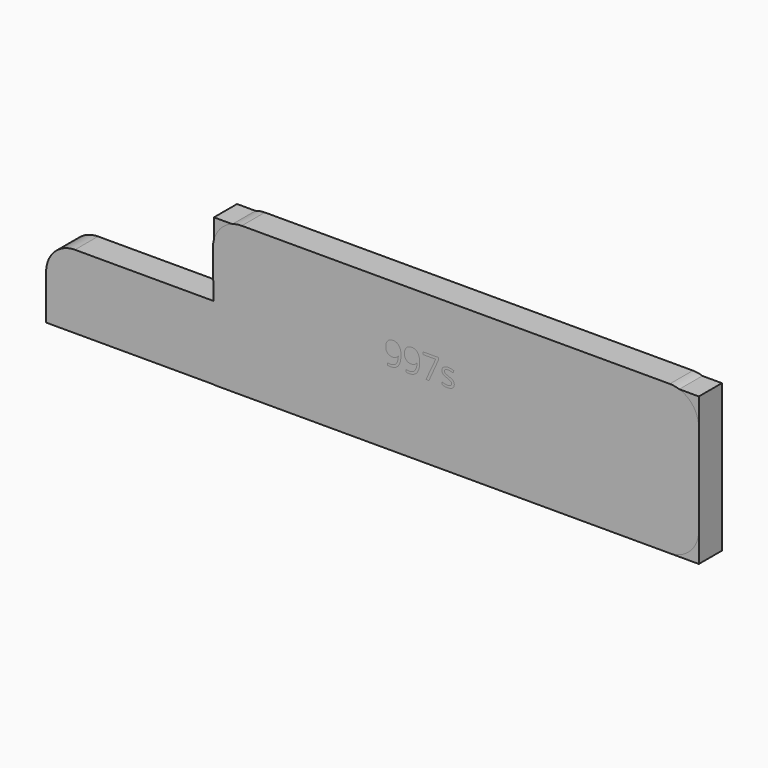
from build123d import *

# Parameters (mm, degrees)
F0_W     = 106.6769063473
F0_H     = 32.4518792331
F0_R     = 4.3257517809
F0_R_2   = 4.488024189
F3_DEPTH = 3.175
F2_R     = 3.175


# Not quite as in the source:
# - a feature of the source that left no trace in its solid (it failed there, or was rolled back) is left out


with BuildPart() as f3:
    # F0 (on Front) → F3 (new body, symmetric)
    with BuildSketch(Plane.XZ):
        Rectangle(F0_W, F0_H)
        with Locations((-36.4220477641, 0)):
            Circle(F0_R, mode=Mode.SUBTRACT)
        with Locations((28.4816995263, 0)):
            Circle(F0_R_2, mode=Mode.SUBTRACT)
    extrude(amount=F3_DEPTH, both=True)


with BuildPart() as f3b:
    # F2 (on Front) → F3, piece 2 (new body, symmetric)
    with BuildSketch(Plane.XZ):
        with Locations((-64.5567512191, -7.0469792688)):
            Circle(F2_R)
    extrude(amount=F3_DEPTH, both=True)


with BuildPart() as f3c:
    # F2 (on Front) → F3, piece 3 (new body, symmetric)
    with BuildSketch(Plane.XZ):
        with Locations((-81.8562208981, -7.2605534128)):
            Circle(F2_R)
    extrude(amount=F3_DEPTH, both=True)


with BuildPart() as f3d:
    # F1 (on Front) → F3, piece 4 (new body, symmetric)
    with BuildSketch(Plane.XZ):
        with BuildLine():
            Line((-53.5699327432, 10.1530148363), (-53.443018347, 0))
            Line((-53.443018347, 0), (-83.9200959526, 0))
            ThreePointArc((-83.9200959526, 0), (-88.4102240131, -1.8598719395), (-90.2700959526, -6.35))
            Line((-90.2700959526, -6.35), (-90.2700959526, -16.1678250879))
            Line((-90.2700959526, -16.1678250879), (-53.443018347, -16.1678250879))
            Line((-53.443018347, -16.1678250879), (46.9560766757, -16.1678250879))
            ThreePointArc((46.9560766757, -16.1678250879), (51.4462047362, -14.3079531484), (53.3060766757, -9.8178250879))
            Line((53.3060766757, -9.8178250879), (53.3060766757, 10.2323847055))
            ThreePointArc((53.3060766757, 10.2323847055), (51.4462047362, 14.7225127661), (46.9560766757, 16.5823847055))
            Line((46.9560766757, 16.5823847055), (-47.2204287922, 16.5823847055))
            ThreePointArc((-47.2204287922, 16.5823847055), (-51.7385311963, 14.6943630409), (-53.5699327432, 10.1530148363))
        make_face()
        with BuildLine():
            add(Edge.make_bspline(
                [(-0.7073512806, 1.6868472509), (-0.4666944061, 1.4338201633), (-0.4666944061, 1.0503435549)],
                knots=[0, 0, 0, 1, 1, 1], degree=2))
            add(Edge.make_bspline(
                [(-0.4666944061, 1.0503435549), (-0.4666944061, 0.5128015643), (-0.867039487, 0.2209769899)],
                knots=[0, 0, 0, 1, 1, 1], degree=2))
            add(Edge.make_bspline(
                [(-0.867039487, 0.2209769899), (-1.2673845679, -0.0708475845), (-1.9916043209, -0.0708475845)],
                knots=[0, 0, 0, 1, 1, 1], degree=2))
            add(Edge.make_bspline(
                [(-1.9916043209, -0.0708475845), (-2.7574329728, -0.0708475845), (-3.1858921746, 0.1720584196)],
                knots=[0, 0, 0, 1, 1, 1], degree=2))
            Line((-3.1858921746, 0.1720584196), (-3.1858921746, 0.7129741047))
            add(Edge.make_bspline(
                [(-3.1858921746, 0.7129741047), (-2.9081246606, 0.5724035005), (-2.590435095, 0.4919971149)],
                knots=[0, 0, 0, 1, 1, 1], degree=2))
            add(Edge.make_bspline(
                [(-2.590435095, 0.4919971149), (-2.2727455294, 0.4115907292), (-1.9769849781, 0.4115907292)],
                knots=[0, 0, 0, 1, 1, 1], degree=2))
            add(Edge.make_bspline(
                [(-1.9769849781, 0.4115907292), (-1.5204116555, 0.4115907292), (-1.2746942393, 0.5572218752)],
                knots=[0, 0, 0, 1, 1, 1], degree=2))
            add(Edge.make_bspline(
                [(-1.2746942393, 0.5572218752), (-1.0289768231, 0.7028530212), (-1.0289768231, 1.001987267)],
                knots=[0, 0, 0, 1, 1, 1], degree=2))
            add(Edge.make_bspline(
                [(-1.0289768231, 1.001987267), (-1.0289768231, 1.2269002338), (-1.2235265393, 1.3865884403)],
                knots=[0, 0, 0, 1, 1, 1], degree=2))
            add(Edge.make_bspline(
                [(-1.2235265393, 1.3865884403), (-1.4180762556, 1.5462766467), (-1.9848569319, 1.7644422245)],
                knots=[0, 0, 0, 1, 1, 1], degree=2))
            add(Edge.make_bspline(
                [(-1.9848569319, 1.7644422245), (-2.5223989225, 1.9646147649), (-2.7489987366, 2.1141818878)],
                knots=[0, 0, 0, 1, 1, 1], degree=2))
            add(Edge.make_bspline(
                [(-2.7489987366, 2.1141818878), (-2.9755985506, 2.2637490107), (-3.0863681868, 2.4532381853)],
                knots=[0, 0, 0, 1, 1, 1], degree=2))
            add(Edge.make_bspline(
                [(-3.0863681868, 2.4532381853), (-3.1971378229, 2.6427273598), (-3.1971378229, 2.9058755309)],
                knots=[0, 0, 0, 1, 1, 1], degree=2))
            add(Edge.make_bspline(
                [(-3.1971378229, 2.9058755309), (-3.1971378229, 3.3770681963), (-2.8136612145, 3.6497751686)],
                knots=[0, 0, 0, 1, 1, 1], degree=2))
            add(Edge.make_bspline(
                [(-2.8136612145, 3.6497751686), (-2.4301846062, 3.9224821408), (-1.7633176596, 3.9224821408)],
                knots=[0, 0, 0, 1, 1, 1], degree=2))
            add(Edge.make_bspline(
                [(-1.7633176596, 3.9224821408), (-1.1414333065, 3.9224821408), (-0.5465385093, 3.6694550532)],
                knots=[0, 0, 0, 1, 1, 1], degree=2))
            Line((-0.5465385093, 3.6694550532), (-0.7545830036, 3.1948886932))
            add(Edge.make_bspline(
                [(-0.7545830036, 3.1948886932), (-1.3337338931, 3.433296438), (-1.8049265585, 3.433296438)],
                knots=[0, 0, 0, 1, 1, 1], degree=2))
            add(Edge.make_bspline(
                [(-1.8049265585, 3.433296438), (-2.2198909822, 3.433296438), (-2.4307468886, 3.3034091997)],
                knots=[0, 0, 0, 1, 1, 1], degree=2))
            add(Edge.make_bspline(
                [(-2.4307468886, 3.3034091997), (-2.6416027949, 3.1735219614), (-2.6416027949, 2.9452353001)],
                knots=[0, 0, 0, 1, 1, 1], degree=2))
            add(Edge.make_bspline(
                [(-2.6416027949, 2.9452353001), (-2.6416027949, 2.790045353), (-2.5623209741, 2.6815248465)],
                knots=[0, 0, 0, 1, 1, 1], degree=2))
            add(Edge.make_bspline(
                [(-2.5623209741, 2.6815248465), (-2.4830391534, 2.5730043401), (-2.3076070393, 2.4746049171)],
                knots=[0, 0, 0, 1, 1, 1], degree=2))
            add(Edge.make_bspline(
                [(-2.3076070393, 2.4746049171), (-2.1321749252, 2.3762054941), (-1.6328681389, 2.1895277317)],
                knots=[0, 0, 0, 1, 1, 1], degree=2))
            add(Edge.make_bspline(
                [(-1.6328681389, 2.1895277317), (-0.948008155, 1.9398743386), (-0.7073512806, 1.6868472509)],
                knots=[0, 0, 0, 1, 1, 1], degree=2))
        make_face(mode=Mode.SUBTRACT)
        with BuildLine():
            add(Edge.make_bspline(
                [(-12.3955158822, 4.1592030383), (-12.1846599758, 3.6447146268), (-12.1846599758, 2.9452353001)],
                knots=[0, 0, 0, 1, 1, 1], degree=2))
            add(Edge.make_bspline(
                [(-12.1846599758, 2.9452353001), (-12.1846599758, -0.0708475845), (-14.5181320062, -0.0708475845)],
                knots=[0, 0, 0, 1, 1, 1], degree=2))
            add(Edge.make_bspline(
                [(-14.5181320062, -0.0708475845), (-14.926349041, -0.0708475845), (-15.1647567858, 0)],
                knots=[0, 0, 0, 1, 1, 1], degree=2))
            Line((-15.1647567858, 0), (-15.1647567858, 0.5026804808))
            add(Edge.make_bspline(
                [(-15.1647567858, 0.5026804808), (-14.8836155773, 0.4115907292), (-14.5260039601, 0.4115907292)],
                knots=[0, 0, 0, 1, 1, 1], degree=2))
            add(Edge.make_bspline(
                [(-14.5260039601, 0.4115907292), (-13.6825803346, 0.4115907292), (-13.2518720032, 0.9333888122)],
                knots=[0, 0, 0, 1, 1, 1], degree=2))
            add(Edge.make_bspline(
                [(-13.2518720032, 0.9333888122), (-12.8211636718, 1.4551868951), (-12.7829284675, 2.5336445709)],
                knots=[0, 0, 0, 1, 1, 1], degree=2))
            Line((-12.7829284675, 2.5336445709), (-12.8245373663, 2.5336445709))
            add(Edge.make_bspline(
                [(-12.8245373663, 2.5336445709), (-13.0179625178, 2.2423822789), (-13.337901213, 2.0894414615)],
                knots=[0, 0, 0, 1, 1, 1], degree=2))
            add(Edge.make_bspline(
                [(-13.337901213, 2.0894414615), (-13.6578399083, 1.9365006441), (-14.0581849892, 1.9365006441)],
                knots=[0, 0, 0, 1, 1, 1], degree=2))
            add(Edge.make_bspline(
                [(-14.0581849892, 1.9365006441), (-14.7396712785, 1.9365006441), (-15.1405786418, 2.3441553964)],
                knots=[0, 0, 0, 1, 1, 1], degree=2))
            add(Edge.make_bspline(
                [(-15.1405786418, 2.3441553964), (-15.5414860051, 2.7518101487), (-15.5414860051, 3.4827772907)],
                knots=[0, 0, 0, 1, 1, 1], degree=2))
            add(Edge.make_bspline(
                [(-15.5414860051, 3.4827772907), (-15.5414860051, 4.2834674525), (-15.0933469188, 4.7473504465)],
                knots=[0, 0, 0, 1, 1, 1], degree=2))
            add(Edge.make_bspline(
                [(-15.0933469188, 4.7473504465), (-14.6452078325, 5.2112334405), (-13.9142406904, 5.2112334405)],
                knots=[0, 0, 0, 1, 1, 1], degree=2))
            add(Edge.make_bspline(
                [(-13.9142406904, 5.2112334405), (-13.3901934778, 5.2112334405), (-12.9982826332, 4.9424624452)],
                knots=[0, 0, 0, 1, 1, 1], degree=2))
            add(Edge.make_bspline(
                [(-12.9982826332, 4.9424624452), (-12.6063717885, 4.6736914499), (-12.3955158822, 4.1592030383)],
                knots=[0, 0, 0, 1, 1, 1], degree=2))
        make_face(mode=Mode.SUBTRACT)
        with BuildLine():
            add(Edge.make_bspline(
                [(-8.2807331548, 4.1592030383), (-8.0698772484, 3.6447146268), (-8.0698772484, 2.9452353001)],
                knots=[0, 0, 0, 1, 1, 1], degree=2))
            add(Edge.make_bspline(
                [(-8.0698772484, 2.9452353001), (-8.0698772484, -0.0708475845), (-10.4033492788, -0.0708475845)],
                knots=[0, 0, 0, 1, 1, 1], degree=2))
            add(Edge.make_bspline(
                [(-10.4033492788, -0.0708475845), (-10.8115663136, -0.0708475845), (-11.0499740583, 0)],
                knots=[0, 0, 0, 1, 1, 1], degree=2))
            Line((-11.0499740583, 0), (-11.0499740583, 0.5026804808))
            add(Edge.make_bspline(
                [(-11.0499740583, 0.5026804808), (-10.7688328499, 0.4115907292), (-10.4112212327, 0.4115907292)],
                knots=[0, 0, 0, 1, 1, 1], degree=2))
            add(Edge.make_bspline(
                [(-10.4112212327, 0.4115907292), (-9.5677976072, 0.4115907292), (-9.1370892758, 0.9333888122)],
                knots=[0, 0, 0, 1, 1, 1], degree=2))
            add(Edge.make_bspline(
                [(-9.1370892758, 0.9333888122), (-8.7063809444, 1.4551868951), (-8.6681457401, 2.5336445709)],
                knots=[0, 0, 0, 1, 1, 1], degree=2))
            Line((-8.6681457401, 2.5336445709), (-8.7097546389, 2.5336445709))
            add(Edge.make_bspline(
                [(-8.7097546389, 2.5336445709), (-8.9031797903, 2.2423822789), (-9.2231184856, 2.0894414615)],
                knots=[0, 0, 0, 1, 1, 1], degree=2))
            add(Edge.make_bspline(
                [(-9.2231184856, 2.0894414615), (-9.5430571809, 1.9365006441), (-9.9434022617, 1.9365006441)],
                knots=[0, 0, 0, 1, 1, 1], degree=2))
            add(Edge.make_bspline(
                [(-9.9434022617, 1.9365006441), (-10.6248885511, 1.9365006441), (-11.0257959144, 2.3441553964)],
                knots=[0, 0, 0, 1, 1, 1], degree=2))
            add(Edge.make_bspline(
                [(-11.0257959144, 2.3441553964), (-11.4267032777, 2.7518101487), (-11.4267032777, 3.4827772907)],
                knots=[0, 0, 0, 1, 1, 1], degree=2))
            add(Edge.make_bspline(
                [(-11.4267032777, 3.4827772907), (-11.4267032777, 4.2834674525), (-10.9785641914, 4.7473504465)],
                knots=[0, 0, 0, 1, 1, 1], degree=2))
            add(Edge.make_bspline(
                [(-10.9785641914, 4.7473504465), (-10.5304251051, 5.2112334405), (-9.799457963, 5.2112334405)],
                knots=[0, 0, 0, 1, 1, 1], degree=2))
            add(Edge.make_bspline(
                [(-9.799457963, 5.2112334405), (-9.2754107504, 5.2112334405), (-8.8834999058, 4.9424624452)],
                knots=[0, 0, 0, 1, 1, 1], degree=2))
            add(Edge.make_bspline(
                [(-8.8834999058, 4.9424624452), (-8.4915890611, 4.6736914499), (-8.2807331548, 4.1592030383)],
                knots=[0, 0, 0, 1, 1, 1], degree=2))
        make_face(mode=Mode.SUBTRACT)
        Polygon((-6.0355394638, 0), (-6.6821642433, 0), (-4.5533630126, 4.6005947357), (-7.3535294492, 4.6005947357), (-7.3535294492, 5.1381367263), (-3.934852354, 5.1381367263), (-3.934852354, 4.6703177554), align=None, mode=Mode.SUBTRACT)
    extrude(amount=F3_DEPTH, both=True)


solid = Compound([f3.part, f3b.part, f3c.part, f3d.part])
